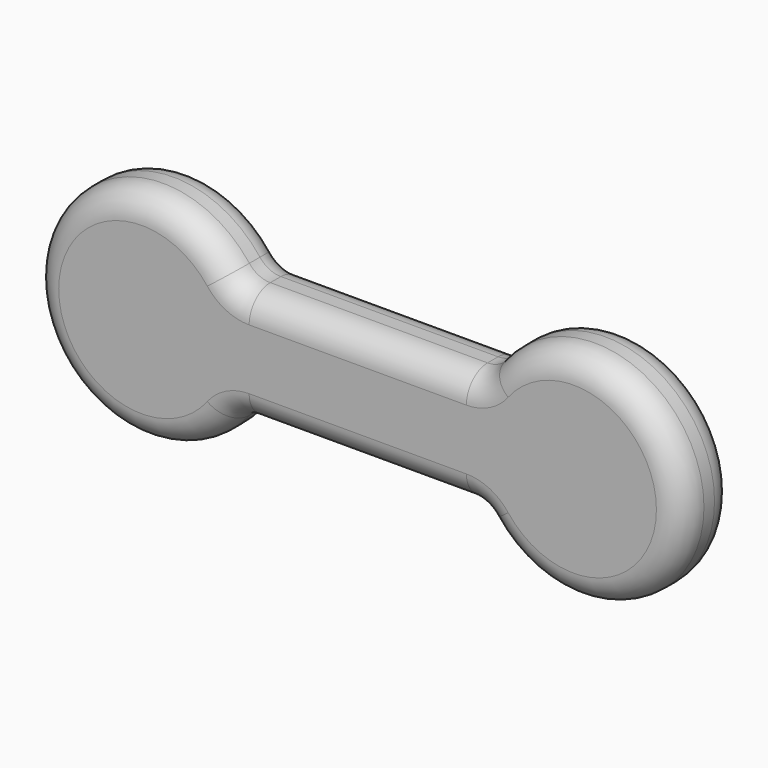
from build123d import *

# Parameters (mm, degrees)
F1_DEPTH = 12.7
F2_R     = 5.08


with BuildPart() as f1:
    # F0 (on Front) → F1 (new body)
    with BuildSketch(Plane.XZ):
        with BuildLine():
            Line((-28.5442825407, -19.2357096821), (-15.6568741476, -19.2357096821))
            ThreePointArc((-15.6568741476, -19.2357096821), (-54.678540264, -30.1371803507), (-15.6568741476, -41.0386510193))
            Line((-15.6568741476, -41.0386510193), (-28.5442825407, -41.0386510193))
            Line((-28.5442825407, -41.0386510193), (-28.5442825407, -19.2357096821))
        make_face()
        with BuildLine():
            Line((42.9155228194, -41.0386510193), (42.9155228194, -19.2357096821))
            Line((42.9155228194, -19.2357096821), (31.4341556288, -19.2357096821))
            ThreePointArc((31.4341556288, -19.2357096821), (28.3832827885, -30.1371803507), (31.4341556288, -41.0386510193))
            Line((31.4341556288, -41.0386510193), (42.9155228194, -41.0386510193))
        make_face()
        with BuildLine():
            ThreePointArc((31.4341556288, -41.0386510193), (28.3832827885, -30.1371803507), (31.4341556288, -19.2357096821))
            Line((31.4341556288, -19.2357096821), (-15.6568741476, -19.2357096821))
            ThreePointArc((-15.6568741476, -19.2357096821), (-13.3870219255, -24.4777329529), (-12.6113336936, -30.1371803507))
            ThreePointArc((-12.6113336936, -30.1371803507), (-13.3870219255, -35.7966277486), (-15.6568741476, -41.0386510193))
            Line((-15.6568741476, -41.0386510193), (31.4341556288, -41.0386510193))
        make_face()
        with BuildLine():
            ThreePointArc((-12.6113336936, -30.1371803507), (-13.3870219255, -24.4777329529), (-15.6568741476, -19.2357096821))
            Line((-15.6568741476, -19.2357096821), (-28.5442825407, -19.2357096821))
            Line((-28.5442825407, -19.2357096821), (-28.5442825407, -41.0386510193))
            Line((-28.5442825407, -41.0386510193), (-15.6568741476, -41.0386510193))
            ThreePointArc((-15.6568741476, -41.0386510193), (-13.3870219255, -35.7966277486), (-12.6113336936, -30.1371803507))
        make_face()
        with BuildLine():
            Line((31.4341556288, -19.2357096821), (42.9155228194, -19.2357096821))
            Line((42.9155228194, -19.2357096821), (42.9155228194, -41.0386510193))
            Line((42.9155228194, -41.0386510193), (31.4341556288, -41.0386510193))
            ThreePointArc((31.4341556288, -41.0386510193), (55.0456161452, -50.3622536115), (70.3876187723, -30.1371803507))
            ThreePointArc((70.3876187723, -30.1371803507), (55.0456161452, -9.91210709), (31.4341556288, -19.2357096821))
        make_face()
    extrude(amount=F1_DEPTH)

    # F2
    f2_edges = [f1.edges().sort_by_distance(p)[0] for p in [
        (-54.67854, 0, -30.13718),
        (-15.656874, -6.35, -19.23571),
        (-15.656874, -6.35, -41.038651),
        (-54.67854, -12.7, -30.13718),
        (7.888641, 0, -41.038651),
        (70.387619, 0, -30.13718),
        (7.888641, 0, -19.23571),
        (31.434156, -6.35, -41.038651),
        (31.434156, -6.35, -19.23571),
        (70.387619, -12.7, -30.13718),
        (7.888641, -12.7, -41.038651),
        (7.888641, -12.7, -19.23571),
    ]]
    fillet(f2_edges, radius=F2_R)


solid = f1.part
